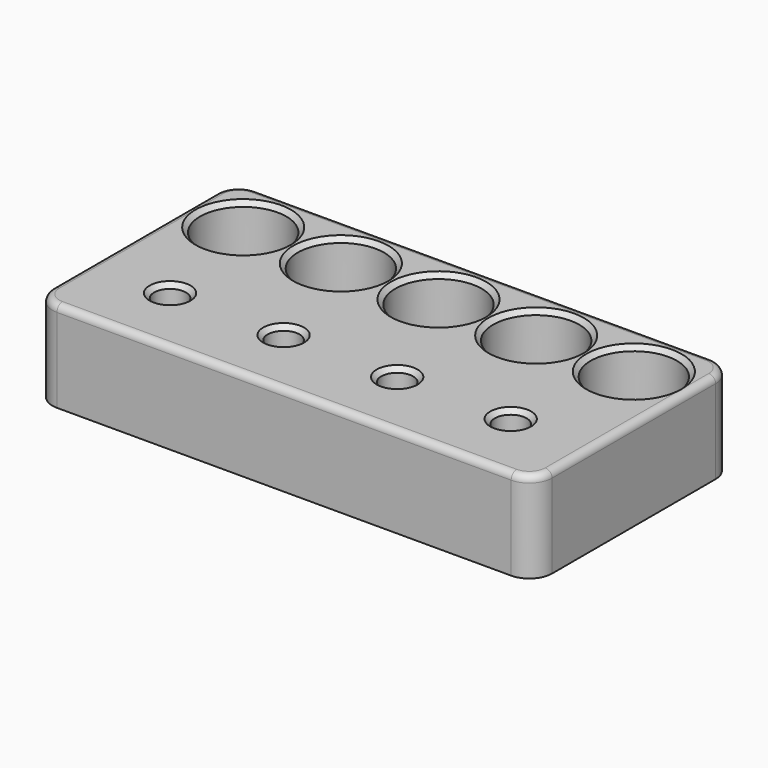
from build123d import *

# Parameters (mm, degrees)
F0_R     = 12.5
F0_R_2   = 9.5
F0_R_3   = 3.5
F1_DEPTH = 20
F2_DEPTH = 5
F3_R     = 1.5
F4_SIZE  = 0.99999
F5_SIZE  = 1


# Not quite as in the source:
# - a fillet or chamfer is up to 0.001 mm smaller than in the source, because OpenCascade refuses the exact size


with BuildPart() as f1:
    # F0 (on Top) → F1 (new body)
    with BuildSketch(Plane.XY):
        with BuildLine():
            Line((50, 27.5), (-50, 27.5))
            ThreePointArc((-50, 27.5), (-53.5355339059, 26.0355339059), (-55, 22.5))
            Line((-55, 22.5), (-55, -22.5))
            ThreePointArc((-55, -22.5), (-53.5355339059, -26.0355339059), (-50, -27.5))
            Line((-50, -27.5), (50, -27.5))
            ThreePointArc((50, -27.5), (53.5355339059, -26.0355339059), (55, -22.5))
            Line((55, -22.5), (55, 22.5))
            ThreePointArc((55, 22.5), (53.5355339059, 26.0355339059), (50, 27.5))
        make_face()
        with Locations((-37.5, -12)):
            Circle(F0_R, mode=Mode.SUBTRACT)
        with BuildLine():
            ThreePointArc((0, -12), (-12.5, -24.5), (-25, -12))
            ThreePointArc((-25, -12), (-12.5, 0.5), (0, -12))
        make_face(mode=Mode.SUBTRACT)
        with BuildLine():
            ThreePointArc((25, -12), (12.5, -24.5), (0, -12))
            ThreePointArc((0, -12), (12.5, 0.5), (25, -12))
        make_face(mode=Mode.SUBTRACT)
        with BuildLine():
            ThreePointArc((50, -12), (37.5, -24.5), (25, -12))
            ThreePointArc((25, -12), (37.5, 0.5), (50, -12))
        make_face(mode=Mode.SUBTRACT)
        with Locations((-43, 15)):
            Circle(F0_R_2, mode=Mode.SUBTRACT)
        with Locations((-21.5, 15)):
            Circle(F0_R_2, mode=Mode.SUBTRACT)
        with Locations((0, 15)):
            Circle(F0_R_2, mode=Mode.SUBTRACT)
        with Locations((21.5, 15)):
            Circle(F0_R_2, mode=Mode.SUBTRACT)
        with Locations((43, 15)):
            Circle(F0_R_2, mode=Mode.SUBTRACT)
        with BuildLine():
            ThreePointArc((0, -12), (-12.5, 0.5), (-25, -12))
            ThreePointArc((-25, -12), (-12.5, -24.5), (0, -12))
        make_face()
        with Locations((-12.5, -12)):
            Circle(F0_R_3, mode=Mode.SUBTRACT)
        with Locations((-37.5, -12)):
            Circle(F0_R)
        with Locations((-37.5, -12)):
            Circle(F0_R_3, mode=Mode.SUBTRACT)
        with BuildLine():
            ThreePointArc((25, -12), (12.5, 0.5), (0, -12))
            ThreePointArc((0, -12), (12.5, -24.5), (25, -12))
        make_face()
        with Locations((12.5, -12)):
            Circle(F0_R_3, mode=Mode.SUBTRACT)
        with BuildLine():
            ThreePointArc((50, -12), (37.5, 0.5), (25, -12))
            ThreePointArc((25, -12), (37.5, -24.5), (50, -12))
        make_face()
        with Locations((37.5, -12)):
            Circle(F0_R_3, mode=Mode.SUBTRACT)
    extrude(amount=F1_DEPTH)

    # F0 (on Top) → F2 (join)
    with BuildSketch(Plane.XY):
        with Locations((-43, 15)):
            Circle(F0_R_2)
        with Locations((-21.5, 15)):
            Circle(F0_R_2)
        with Locations((0, 15)):
            Circle(F0_R_2)
        with Locations((21.5, 15)):
            Circle(F0_R_2)
        with Locations((43, 15)):
            Circle(F0_R_2)
    extrude(amount=F2_DEPTH)

    # F3
    f3_edges = [f1.edges().sort_by_distance(p)[0] for p in [
        (0, -27.5, 20),
    ]]
    fillet(f3_edges, radius=F3_R)

    # F4 (size 1 in the source; OpenCascade refuses exactly that, so slightly less here)
    f4_edges = [f1.edges().sort_by_distance(p)[0] for p in [
        (-52.5, 15, 20),
        (-31, 15, 20),
        (-9.5, 15, 20),
        (12, 15, 20),
        (33.5, 15, 20),
    ]]
    chamfer(f4_edges, length=F4_SIZE)

    # F5
    f5_edges = [f1.edges().sort_by_distance(p)[0] for p in [
        (-41, -12, 20),
        (-16, -12, 20),
        (9, -12, 20),
        (34, -12, 20),
    ]]
    chamfer(f5_edges, length=F5_SIZE)


solid = f1.part
